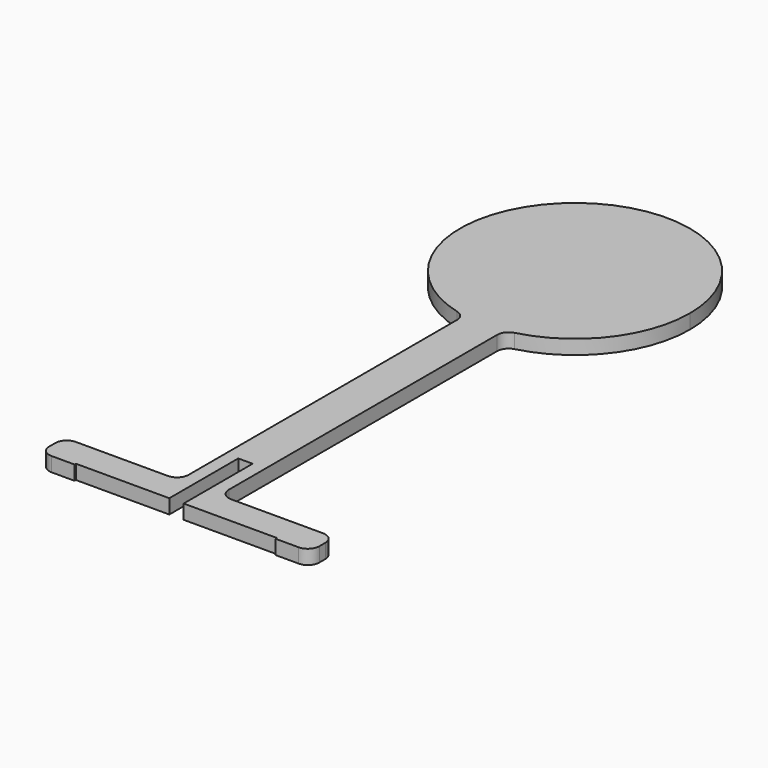
from build123d import *

# Parameters (mm, degrees)
F0_W     = 6
F0_H     = 0.3
F1_DEPTH = 2.5
F2_R     = 2


# Not quite as in the source:
# - a feature names something its author has since deleted; it is built from what else it names


with BuildPart() as f1:
    # F0 (on Top) → F1 (new body)
    with BuildSketch(Plane.XY):
        with BuildLine():
            ThreePointArc((3.5, -3), (0, -3.3086313325), (-3.5, -3))
            Line((-3.5, -3), (-3.5, -65))
            Line((-3.5, -65), (-23.5, -65))
            Line((-23.5, -65), (-23.5, -70))
            Line((-23.5, -70), (-17.5, -70))
            Line((-17.5, -70), (-1.25, -70))
            Line((-1.25, -70), (-1.25, -55))
            Line((-1.25, -55), (1.25, -55))
            Line((1.25, -55), (1.25, -70))
            Line((1.25, -70), (17.5, -70))
            Line((17.5, -70), (23.5, -70))
            Line((23.5, -70), (23.5, -65))
            Line((23.5, -65), (3.5, -65))
            Line((3.5, -65), (3.5, -3))
        make_face()
        with BuildLine():
            ThreePointArc((20, 16.6913686675), (-12.8452325787, 32.0210783843), (-3.5, -3))
            ThreePointArc((-3.5, -3), (0, -3.3086313325), (3.5, -3))
            ThreePointArc((3.5, -3), (15.3297097168, 3.8461360889), (20, 16.6913686675))
        make_face()
        with Locations((-20.5, -70.15)):
            Rectangle(F0_W, F0_H)
        with Locations((20.5, -70.15)):
            Rectangle(F0_W, F0_H)
    extrude(amount=F1_DEPTH)

    # F2
    f2_edges = [f1.edges().sort_by_distance(p)[0] for p in [
        (-3.5, -3, 1.25),
        (3.5, -3, 1.25),
        (23.5, -65, 1.25),
        (-23.5, -65, 1.25),
        (-3.5, -65, 1.25),
        (3.5, -65, 1.25),
        (-23.5, -70.3, 1.25),
        (23.5, -70.3, 1.25),
    ]]
    fillet(f2_edges, radius=F2_R)


solid = f1.part
